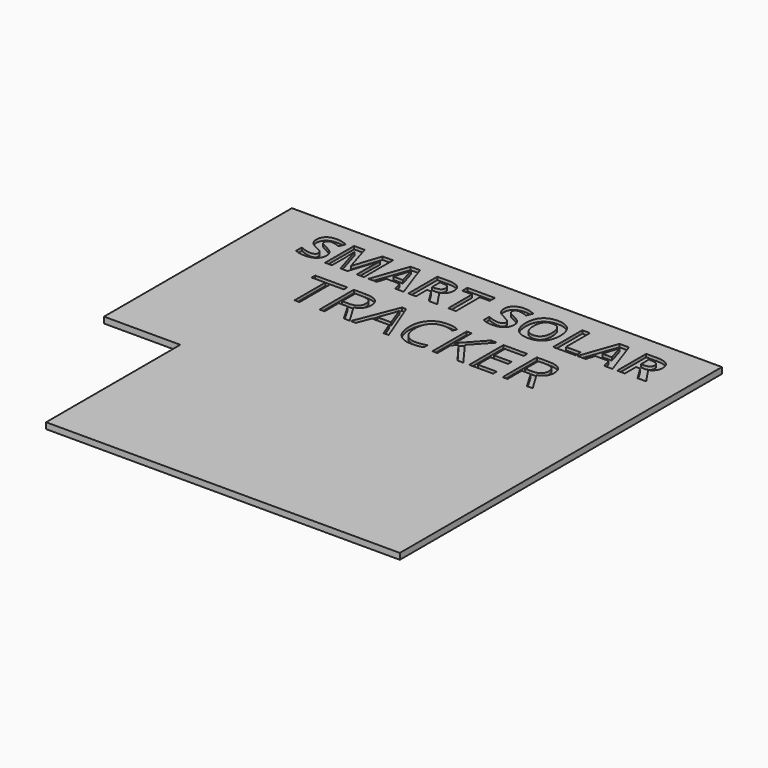
from build123d import *

# Parameters (mm, degrees)
F0_W         = 141
F0_H         = 142
F1_DEPTH     = 2
F2_W         = 25
F2_H         = 50
F3_DEPTH     = 9.5
F4_TEXT_SIZE = 16.7025874058
F5_DEPTH     = 1
F6_TEXT_SIZE = 19.665947184
F7_DEPTH     = 1
F8_W         = 25
F8_H         = 5
F9_DEPTH     = 5
F10_W        = 141
F10_H        = 10
F11_DEPTH    = 3


# Not quite as in the source:
# - Text() gives the source's letters only with a copy of the font that has no kerning and outlines rounded to 1/6400 em; it was checked with that copy


with BuildPart() as f1:
    # F0 (on Top) → F1 (new body)
    with BuildSketch(Plane.XY):
        Rectangle(F0_W, F0_H)
    extrude(amount=F1_DEPTH)

    # F2 (on face) → F3 (cut)
    with BuildSketch(Plane.XY.offset(2)):
        with Locations((-58, -46)):
            Rectangle(F2_W, F2_H)
    extrude(amount=-F3_DEPTH, mode=Mode.SUBTRACT)

    # F4 (on face) → F5 (cut)
    with BuildSketch(Plane.XY.offset(2)):
        with Locations((-55.66810444, 42.6724180579)):
            Text('SMART SOLAR', F4_TEXT_SIZE, font='Open Sans', font_style=FontStyle.BOLD, text_align=(TextAlign.LEFT, TextAlign.BOTTOM))
    extrude(amount=-F5_DEPTH, mode=Mode.SUBTRACT)

    # F6 (on face) → F7 (cut)
    with BuildSketch(Plane.XY.offset(2)):
        with Locations((-42.6724199206, 21.5301718563)):
            Text('TRACKER', F6_TEXT_SIZE, font='Open Sans', text_align=(TextAlign.LEFT, TextAlign.BOTTOM))
    extrude(amount=-F7_DEPTH, mode=Mode.SUBTRACT)

    # F8 (on face) → F9 (cut)
    with BuildSketch(Plane.XY.offset(2)):
        with Locations((-58, -18.5)):
            Rectangle(F8_W, F8_H)
    extrude(amount=-F9_DEPTH, mode=Mode.SUBTRACT)

    # F10 (on face) → F11 (cut)
    with BuildSketch(Plane.XY.offset(2)):
        with Locations((0, 66)):
            Rectangle(F10_W, F10_H)
    extrude(amount=-F11_DEPTH, mode=Mode.SUBTRACT)


solid = f1.part
